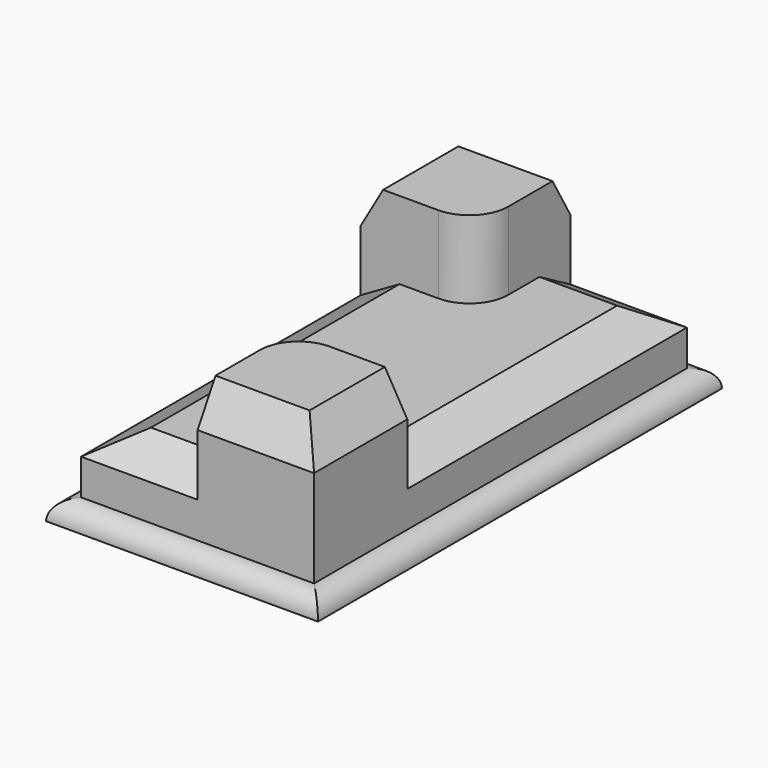
from build123d import *

# Parameters (mm, degrees)
F0_W     = 88.9
F0_H     = 165.1
F1_DEPTH = 6.35
F2_DEPTH = 25.4
F3_DEPTH = 50.8
F4_SIZE2 = 7.3323484187
F4_SIZE  = 12.7
F5_R     = 6.34999
F6_SIZE2 = 7.3323484187
F6_SIZE  = 12.7
F7_SIZE2 = 7.3323484187
F7_SIZE  = 12.7


# Not quite as in the source:
# - a fillet or chamfer is up to 0.001 mm smaller than in the source, because OpenCascade refuses the exact size


with BuildPart() as f1:
    # F0 (on Top) → F1 (new body)
    with BuildSketch(Plane.XY):
        Rectangle(F0_W, F0_H)
        Polygon((-38.1, 38.1), (-38.1, 76.2), (0, 76.2), (38.1, 76.2), (38.1, -38.1), (38.1, -76.2), (0, -76.2), (-38.1, -76.2), align=None, mode=Mode.SUBTRACT)
    extrude(amount=F1_DEPTH)

    # F0 (on Top) → F2 (join)
    with BuildSketch(Plane.XY):
        with BuildLine():
            Line((38.1, 76.2), (0, 76.2))
            Line((0, 76.2), (0, 50.8))
            ThreePointArc((0, 50.8), (-3.7197438789, 41.8197438789), (-12.7, 38.1))
            Line((-12.7, 38.1), (-38.1, 38.1))
            Line((-38.1, 38.1), (-38.1, -76.2))
            Line((-38.1, -76.2), (0, -76.2))
            Line((0, -76.2), (0, -50.8))
            ThreePointArc((0, -50.8), (3.7197438789, -41.8197438789), (12.7, -38.1))
            Line((12.7, -38.1), (38.1, -38.1))
            Line((38.1, -38.1), (38.1, 76.2))
        make_face()
    extrude(amount=F2_DEPTH)

    # F0 (on Top) → F3 (join)
    with BuildSketch(Plane.XY):
        with BuildLine():
            Line((0, 76.2), (-38.1, 76.2))
            Line((-38.1, 76.2), (-38.1, 38.1))
            Line((-38.1, 38.1), (-12.7, 38.1))
            ThreePointArc((-12.7, 38.1), (-3.7197438789, 41.8197438789), (0, 50.8))
            Line((0, 50.8), (0, 76.2))
        make_face()
        with BuildLine():
            Line((38.1, -76.2), (38.1, -38.1))
            Line((38.1, -38.1), (12.7, -38.1))
            ThreePointArc((12.7, -38.1), (3.7197438789, -41.8197438789), (0, -50.8))
            Line((0, -50.8), (0, -76.2))
            Line((0, -76.2), (38.1, -76.2))
        make_face()
    extrude(amount=F3_DEPTH)

    # F4
    f4_edges = [f1.edges().sort_by_distance(p)[0] for p in [
        (-38.1, -19.05, 25.4),
        (-19.05, -76.2, 25.4),
        (38.1, 19.05, 25.4),
        (19.05, 76.2, 25.4),
    ]]
    f4_side = f1.faces().sort_by_distance((0, 0, 25.4))[0]
    chamfer(f4_edges, length=F4_SIZE, length2=F4_SIZE2, reference=f4_side)

    # F5 (radius 6.35 in the source; OpenCascade refuses exactly that, so slightly less here)
    f5_edges = [f1.edges().sort_by_distance(p)[0] for p in [
        (44.45, 0, 6.35),
        (0, -82.55, 6.35),
        (-44.45, 0, 6.35),
        (0, 82.55, 6.35),
    ]]
    fillet(f5_edges, radius=F5_R)

    # F6
    f6_edges = [f1.edges().sort_by_distance(p)[0] for p in [
        (-19.05, 76.2, 50.8),
        (-38.1, 57.15, 50.8),
    ]]
    chamfer(f6_edges, length=F6_SIZE, length2=F6_SIZE2)

    # F7
    f7_edges = [f1.edges().sort_by_distance(p)[0] for p in [
        (38.1, -57.15, 50.8),
        (19.05, -76.2, 50.8),
    ]]
    chamfer(f7_edges, length=F7_SIZE, length2=F7_SIZE2)


solid = f1.part
